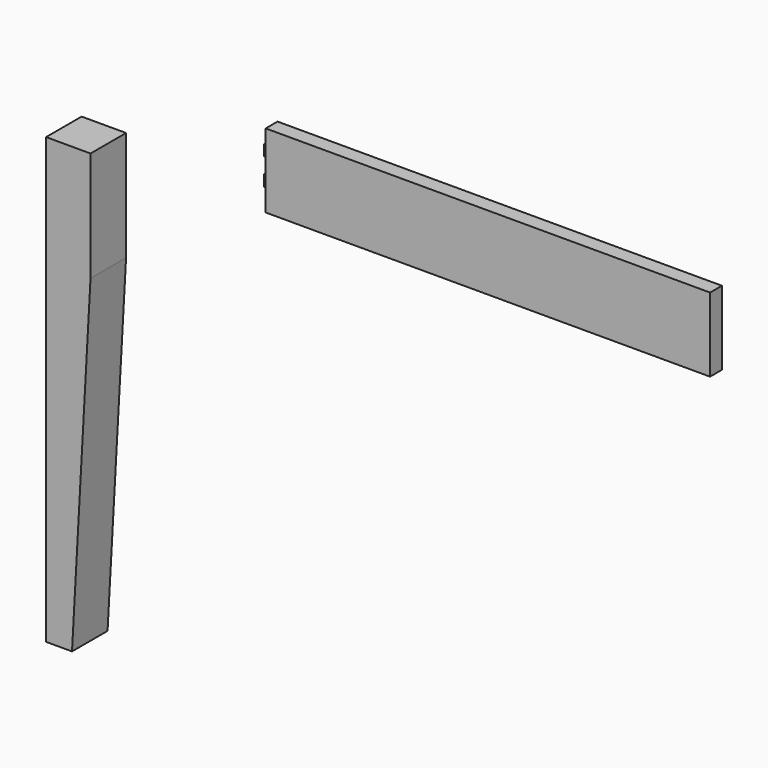
from build123d import *

# Parameters (mm, degrees)
F1_DEPTH  = 60
F3_W      = 600
F3_H      = 100
F4_DEPTH  = 20
F6_DEPTH  = 3
F7_DEPTH  = 3
F8_R      = 1.4141506132
F8_R_2    = 1.3029129936
F8_R_3    = 1.1770229145
F9_DEPTH  = 15
F10_W     = 2.8019864112
F10_H     = 14.732837677
F11_DEPTH = 6
F10_W_2   = 3.2857935876
F10_H_2   = 15.1772499084
F12_DEPTH = 6
F13_W     = 3.067890475
F13_H     = 8.4506869316
F14_DEPTH = 25.4
F15_W     = 3.4896529414
F15_H     = 9.1037750244
F16_DEPTH = 25.4


with BuildPart() as f1:
    # F0 (on Front) → F1 (new body)
    with BuildSketch(Plane.XZ):
        Polygon((0, 600), (0, 0), (35, 0), (60, 451.6516281811), (60, 600), align=None)
    extrude(amount=F1_DEPTH)


with BuildPart() as f4:
    # F3 (on face) → F4 (new body)
    with BuildSketch(Plane.XZ):
        with Locations((564.5029609896, 630.087941885)):
            Rectangle(F3_W, F3_H)
    extrude(amount=F4_DEPTH)

    # F5 (on face) → F6 (cut)
    with BuildSketch(Plane(origin=(264.5029609896, 0, 0), x_dir=(0, -1, 0), z_dir=(-1, 0, 0))):
        with BuildLine():
            ThreePointArc((13.9291705564, 667.7783727646), (9.8136605229, 671.893882798), (5.6981504895, 667.7783727646))
            Line((5.6981504895, 667.7783727646), (5.6981504895, 591.1698937416))
            ThreePointArc((5.6981504895, 591.1698937416), (9.8136605229, 587.0543837082), (13.9291705564, 591.1698937416))
            Line((13.9291705564, 591.1698937416), (13.9291705564, 667.7783727646))
        make_face()
    extrude(amount=-F6_DEPTH, mode=Mode.SUBTRACT)


with BuildPart() as f7:
    # F5 (on face) → F7 (new body)
    with BuildSketch(Plane(origin=(264.5029609896, 0, 0), x_dir=(0, -1, 0), z_dir=(-1, 0, 0))):
        with BuildLine():
            ThreePointArc((13.9291705564, 667.7783727646), (9.8136605229, 671.893882798), (5.6981504895, 667.7783727646))
            Line((5.6981504895, 667.7783727646), (5.6981504895, 591.1698937416))
            ThreePointArc((5.6981504895, 591.1698937416), (9.8136605229, 587.0543837082), (13.9291705564, 591.1698937416))
            Line((13.9291705564, 591.1698937416), (13.9291705564, 667.7783727646))
        make_face()
    extrude(amount=F7_DEPTH)

    # F8 (on face) → F9 (cut)
    with BuildSketch(Plane(origin=(261.5029609896, 0, 0), x_dir=(0, -1, 0), z_dir=(-1, 0, 0))):
        with Locations((9.8758814856, 597.0197916031)):
            Circle(F8_R)
        with Locations((9.8758814856, 664.9664640427)):
            Circle(F8_R_2)
        with Locations((9.8136605229, 629.4741332531)):
            Circle(F8_R_3)
    extrude(amount=-F9_DEPTH, mode=Mode.SUBTRACT)

    # F10 (on face) → F11 (join)
    with BuildSketch(Plane(origin=(261.5029609896, 0, 0), x_dir=(0, -1, 0), z_dir=(-1, 0, 0))):
        with Locations((10.0416680798, 647.6745605469)):
            Rectangle(F10_W, F10_H)
    extrude(amount=F11_DEPTH)

    # F10 (on face) → F12 (join)
    with BuildSketch(Plane(origin=(261.5029609896, 0, 0), x_dir=(0, -1, 0), z_dir=(-1, 0, 0))):
        with Locations((10.0818593055, 611.8075251579)):
            Rectangle(F10_W_2, F10_H_2)
    extrude(amount=F12_DEPTH)

    # F13 (on face) → F14 (cut)
    with BuildSketch(Plane(origin=(0, -8.6406748742, 0), x_dir=(-1, 0, 0), z_dir=(0, 1, 0))):
        with Locations((-259.9690157522, 644.5334851742)):
            Rectangle(F13_W, F13_H)
    extrude(amount=-F14_DEPTH, mode=Mode.SUBTRACT)

    # F15 (on face) → F16 (cut)
    with BuildSketch(Plane(origin=(0, -8.4389625117, 0), x_dir=(-1, 0, 0), z_dir=(0, 1, 0))):
        with Locations((-259.7581345189, 608.7707877159)):
            Rectangle(F15_W, F15_H)
    extrude(amount=-F16_DEPTH, mode=Mode.SUBTRACT)


solid = Compound([f1.part, f4.part, f7.part])
